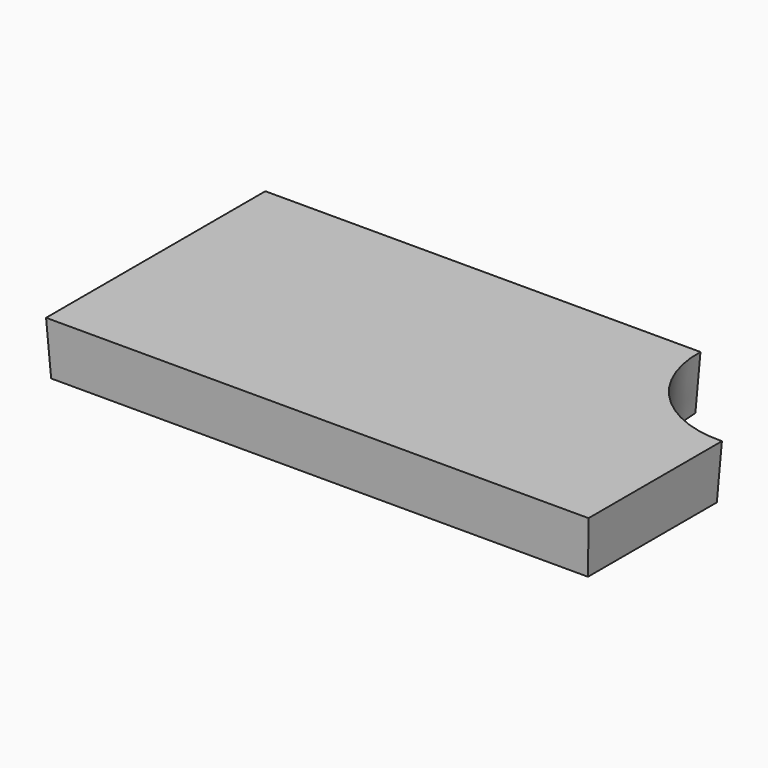
from build123d import *

# Parameters (mm, degrees)
F1_DEPTH               = 25.4
DRAFT_F1_DRAFTED_ANGLE = -3


# Not quite as in the source:
# - an extrude with a draft is written as a straight extrude whose walls are then drafted


with BuildPart() as f1:
    # F0 (on Top) → F1 (new body)
    with BuildSketch(Plane.XY):
        with BuildLine():
            ThreePointArc((127, 12.7), (91.0789755157, 27.5789755157), (76.2, 63.5))
            Line((76.2, 63.5), (-127, 63.5))
            Line((-127, 63.5), (-127, -63.5))
            Line((-127, -63.5), (127, -63.5))
            Line((127, -63.5), (127, 12.7))
        make_face()
    extrude(amount=F1_DEPTH)

    # draft_F1_drafted
    draft_f1_drafted_walls = [f1.faces().sort_by_distance(p)[0] for p in [
        (91.0789755157, 27.5789755157, 16.9333333333),
        (-25.4, 63.5, 16.9333333333),
        (-127, 0, 16.9333333333),
        (0, -63.5, 16.9333333333),
        (127, -25.4, 16.9333333333),
    ]]
    draft(draft_f1_drafted_walls, neutral_plane=Plane.XY, angle=DRAFT_F1_DRAFTED_ANGLE)


solid = f1.part
